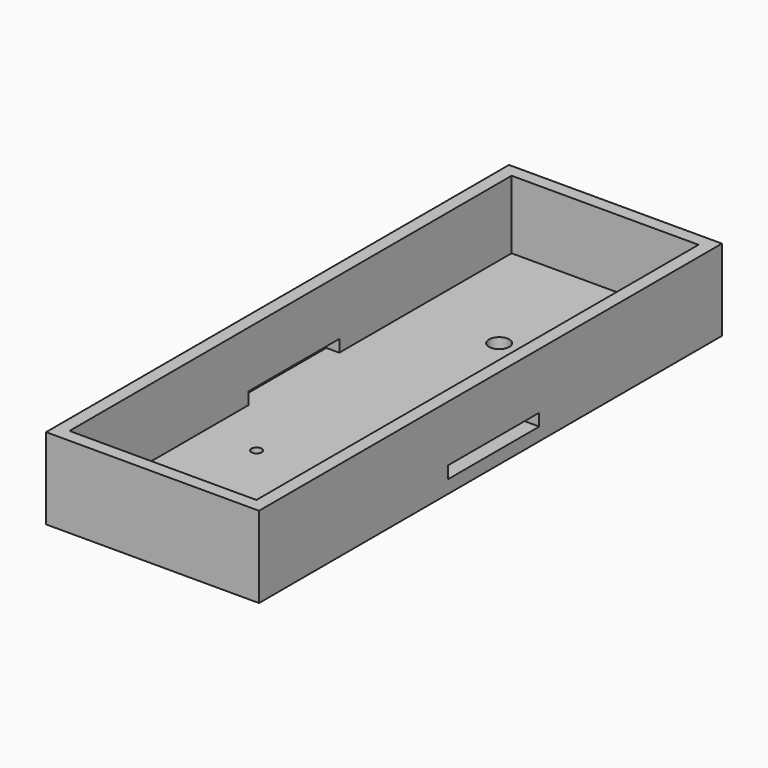
from build123d import *

# Parameters (mm, degrees)
F0_W          = 52.4
F0_H          = 142.4
F0_W_2        = 46
F0_H_2        = 136
F0_R          = 1.25
F0_R_2        = 2.5
F1_DEPTH      = 3.2
F2_DEPTH      = 20
F3_W          = 28
F3_H          = 3
F4_DEPTH      = 3.201
F4_DEPTH_BACK = 49.201


with BuildPart() as f1:
    # F0 (on Top) → F1 (new body)
    with BuildSketch(Plane.XY):
        Rectangle(F0_W, F0_H)
        Rectangle(F0_W_2, F0_H_2, mode=Mode.SUBTRACT)
        Rectangle(F0_W_2, F0_H_2)
        with Locations((-10, -26.7)):
            Circle(F0_R, mode=Mode.SUBTRACT)
        with Locations((10, -26.7)):
            Circle(F0_R, mode=Mode.SUBTRACT)
        with Locations((-1.5, 37.3)):
            Circle(F0_R_2, mode=Mode.SUBTRACT)
    extrude(amount=F1_DEPTH)

    # F0 (on Top) → F2 (join)
    with BuildSketch(Plane.XY):
        Rectangle(F0_W, F0_H)
        Rectangle(F0_W_2, F0_H_2, mode=Mode.SUBTRACT)
    extrude(amount=F2_DEPTH)

    # F3 (on face) → F4 (cut, two sides)
    with BuildSketch(Plane.YZ.offset(-23)) as f4_sk:
        with Locations((1, 4.7)):
            Rectangle(F3_W, F3_H)
    extrude(amount=-F4_DEPTH, mode=Mode.SUBTRACT)
    extrude(f4_sk.sketch, amount=F4_DEPTH_BACK, mode=Mode.SUBTRACT)


solid = f1.part
